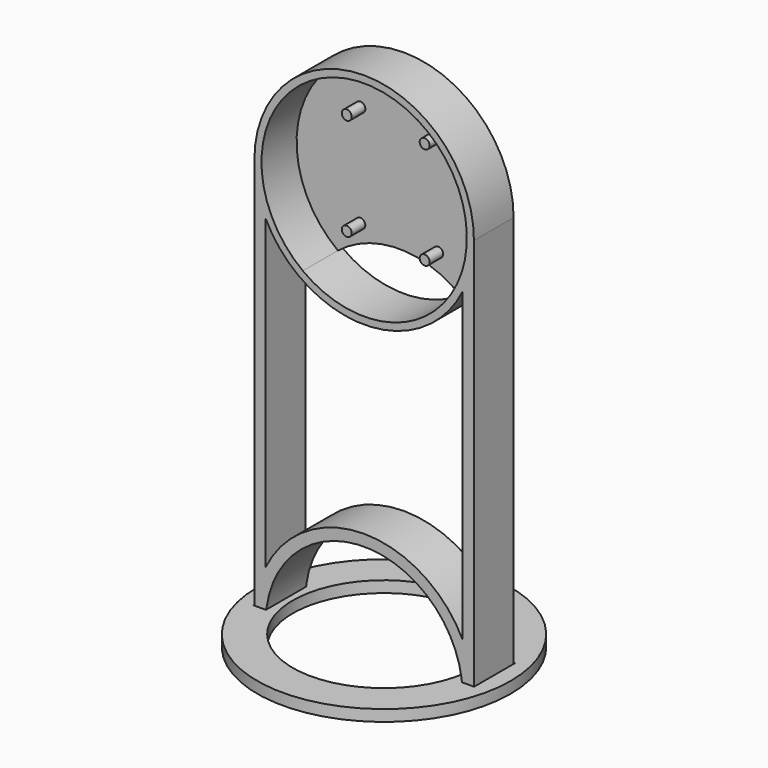
from build123d import *

# Parameters (mm, degrees)
F1_DEPTH    = 14
F0_R        = 1.4
F2_DEPTH    = 1.6
F3_DEPTH    = 6.4
F4_R        = 35.7804971641
F4_W        = 3.6
F4_H        = 14.4
F4_R_2      = 25.7804971641
F5_DEPTH    = 3.2
F8_DEPTH    = 1.6
F9_T1_DEPTH = 3.2
F9_T3_DEPTH = 5.9959172278
F9_T5_DEPTH = 12.5675364253
F10_R       = 0.4


# Not quite as in the source:
# - a fillet or chamfer that OpenCascade refuses, or shapes differently, is made with other operations: its cross-section is extruded or revolved along the edge and cut away or added


with BuildPart() as f1:
    # F0 (on Front) → F1 (new body)
    with BuildSketch(Plane.XZ):
        with BuildLine():
            ThreePointArc((17.3232920146, -23.2573333333), (0, -29), (-17.3232920146, -23.2573333333))
            ThreePointArc((-17.3232920146, -23.2573333333), (-18.1118631329, -23.9097080661), (-18.8758870755, -24.5906666667))
            ThreePointArc((-18.8758870755, -24.5906666667), (0, -31), (18.8758870755, -24.5906666667))
            ThreePointArc((18.8758870755, -24.5906666667), (18.1118631329, -23.9097080661), (17.3232920146, -23.2573333333))
        make_face()
        with BuildLine():
            ThreePointArc((-17.3232920146, -23.2573333333), (-13.0120046799, 25.9169391366), (29, 0))
            ThreePointArc((29, 0), (25.9169391366, -13.0120046799), (17.3232920146, -23.2573333333))
            ThreePointArc((17.3232920146, -23.2573333333), (18.1118631329, -23.9097080661), (18.8758870755, -24.5906666667))
            ThreePointArc((18.8758870755, -24.5906666667), (23.9628460371, -19.6667742602), (27.8, -13.7171425596))
            Line((27.8, -13.7171425596), (27.8, -45))
            Line((27.8, -45), (27.8, -100.2828574404))
            Line((27.8, -100.2828574404), (27.8, -114))
            Line((27.8, -114), (31, -114))
            Line((31, -114), (31, 0))
            ThreePointArc((31, 0), (0, 31), (-31, 0))
            Line((-31, 0), (-31, -114))
            Line((-31, -114), (-27.8, -114))
            Line((-27.8, -114), (-27.8, -100.2828574404))
            Line((-27.8, -100.2828574404), (-27.8, -45))
            Line((-27.8, -45), (-27.8, -13.7171425596))
            ThreePointArc((-27.8, -13.7171425596), (-23.9628460371, -19.6667742602), (-18.8758870755, -24.5906666667))
            ThreePointArc((-18.8758870755, -24.5906666667), (-18.1118631329, -23.9097080661), (-17.3232920146, -23.2573333333))
        make_face()
        with BuildLine():
            ThreePointArc((27.8, -100.2828574404), (0, -83), (-27.8, -100.2828574404))
            Line((-27.8, -100.2828574404), (-27.8, -114))
            ThreePointArc((-27.8, -114), (0, -86.2), (27.8, -114))
            Line((27.8, -114), (27.8, -100.2828574404))
        make_face()
    extrude(amount=F1_DEPTH)

    # F0 (on Front) → F2 (join)
    with BuildSketch(Plane.XZ):
        with BuildLine():
            ThreePointArc((17.3232920146, -23.2573333333), (25.9169391366, -13.0120046799), (29, 0))
            ThreePointArc((29, 0), (-13.0120046799, 25.9169391366), (-17.3232920146, -23.2573333333))
            ThreePointArc((-17.3232920146, -23.2573333333), (0, -17.2), (17.3232920146, -23.2573333333))
        make_face()
        with Locations((-11, -14.45)):
            Circle(F0_R, mode=Mode.SUBTRACT)
        with Locations((-11, 14.45)):
            Circle(F0_R, mode=Mode.SUBTRACT)
        with Locations((11, -14.45)):
            Circle(F0_R, mode=Mode.SUBTRACT)
        with Locations((11, 14.45)):
            Circle(F0_R, mode=Mode.SUBTRACT)
    extrude(amount=F2_DEPTH)

    # F0 (on Front) → F3 (join)
    with BuildSketch(Plane.XZ):
        with Locations((11, -14.45)):
            Circle(F0_R)
        with Locations((-11, -14.45)):
            Circle(F0_R)
        with Locations((-11, 14.45)):
            Circle(F0_R)
        with Locations((11, 14.45)):
            Circle(F0_R)
    extrude(amount=F3_DEPTH)

    # F10
    f10_edges = [f1.edges().sort_by_distance(p)[0] for p in [
        (27.8, -7, -114),
        (31, -7, -114),
        (29.4, -14, -114),
        (29.4, 0, -114),
        (-29.4, 0, -114),
        (-31, -7, -114),
        (-27.8, -7, -114),
        (-29.4, -14, -114),
    ]]
    fillet(f10_edges, radius=F10_R)


with BuildPart() as f5:
    # F4 (on face) → F5 (new body)
    with BuildSketch(Plane(origin=(0, 0, -114), x_dir=(1, 0, 0), z_dir=(0, 0, -1))):
        with Locations((0, 7)):
            Circle(F4_R)
        with Locations((-29.4, 7)):
            Rectangle(F4_W, F4_H, mode=Mode.SUBTRACT)
        with Locations((0, 7)):
            Circle(F4_R_2, mode=Mode.SUBTRACT)
        with Locations((29.4, 7)):
            Rectangle(F4_W, F4_H, mode=Mode.SUBTRACT)
    extrude(amount=-F5_DEPTH)

    # F7 (on offset) → F8 (join, symmetric)
    with BuildSketch(Plane.XZ.offset(-23.2)):
        with BuildLine():
            ThreePointArc((1.5, -107.8606123087), (2.8142494559, -109.076631206), (3.3, -110.8))
            Line((3.3, -110.8), (4.9, -110.8))
            ThreePointArc((4.9, -110.8), (3.9597979746, -107.9138260621), (1.5, -106.1352384841))
            Line((1.5, -106.1352384841), (1.5, -107.8606123087))
        make_face()
        with BuildLine():
            Line((-4.9, -110.8), (-3.3, -110.8))
            ThreePointArc((-3.3, -110.8), (-2.8142494559, -109.076631206), (-1.5, -107.8606123087))
            Line((-1.5, -107.8606123087), (-1.5, -106.1352384841))
            ThreePointArc((-1.5, -106.1352384841), (-3.9597979746, -107.9138260621), (-4.9, -110.8))
        make_face()
    extrude(amount=F8_DEPTH, both=True)

    # F9: fillet of radius 1 on 8 edges, made by hand

    # F9_s2 → F9_t1 (join)
    with BuildSketch(Plane.XZ.offset(-24.8)):
        with BuildLine():
            ThreePointArc((5.814636704, -110.8), (5.1702344715, -110.5646867089), (4.8291050593, -109.9694915254))
            ThreePointArc((4.8291050593, -109.9694915254), (4.8822440942, -110.3832355525), (4.9, -110.8))
            Line((4.9, -110.8), (5.814636704, -110.8))
        make_face()
        with BuildLine():
            ThreePointArc((-5.814636704, -110.8), (-5.1702344715, -110.5646867089), (-4.8291050593, -109.9694915254))
            ThreePointArc((-4.8291050593, -109.9694915254), (-4.8822440942, -110.3832355525), (-4.9, -110.8))
            Line((-4.9, -110.8), (-5.814636704, -110.8))
        make_face()
        with BuildLine():
            ThreePointArc((2.0712315177, -110.8), (2.9182210716, -110.3316095331), (2.9717669602, -109.3652173913))
            ThreePointArc((2.9717669602, -109.3652173913), (3.2168953176, -110.0640757405), (3.3, -110.8))
            Line((3.3, -110.8), (2.0712315177, -110.8))
        make_face()
        with BuildLine():
            ThreePointArc((-2.0712315177, -110.8), (-2.9182210716, -110.3316095331), (-2.9717669602, -109.3652173913))
            ThreePointArc((-2.9717669602, -109.3652173913), (-3.2168953176, -110.0640757405), (-3.3, -110.8))
            Line((-3.3, -110.8), (-2.0712315177, -110.8))
        make_face()
    extrude(amount=F9_T1_DEPTH)

    # F9_s4 → F9_t3 (cut)
    with BuildSketch(Plane.XZ.offset(-26.1979586139)):
        with BuildLine():
            ThreePointArc((1.5, -107.3014288631), (1.6107881724, -107.7589245741), (1.9186046512, -108.1150500577))
            ThreePointArc((1.9186046512, -108.1150500577), (1.7140300704, -107.9800530293), (1.5, -107.8606123087))
            Line((1.5, -107.8606123087), (1.5, -107.3014288631))
        make_face()
        with BuildLine():
            ThreePointArc((-1.5, -107.3014288631), (-1.6107881724, -107.7589245741), (-1.9186046512, -108.1150500577))
            ThreePointArc((-1.9186046512, -108.1150500577), (-1.7140300704, -107.9800530293), (-1.5, -107.8606123087))
            Line((-1.5, -107.8606123087), (-1.5, -107.3014288631))
        make_face()
    extrude(amount=F9_T3_DEPTH, mode=Mode.SUBTRACT)

    # F9_s6 → F9_t5 (cut)
    with BuildSketch(Plane.XZ.offset(-29.4837682127)):
        with BuildLine():
            ThreePointArc((3.141025641, -107.0391546266), (2.0763407271, -106.9008524633), (1.5, -107.8066740906))
            Line((1.5, -107.8066740906), (1.5, -106.1352384841))
            ThreePointArc((1.5, -106.1352384841), (2.3641162933, -106.5080360962), (3.141025641, -107.0391546266))
        make_face()
        with BuildLine():
            ThreePointArc((-3.141025641, -107.0391546266), (-2.0763407271, -106.9008524633), (-1.5, -107.8066740906))
            Line((-1.5, -107.8066740906), (-1.5, -106.1352384841))
            ThreePointArc((-1.5, -106.1352384841), (-2.3641162933, -106.5080360962), (-3.141025641, -107.0391546266))
        make_face()
    extrude(amount=F9_T5_DEPTH, mode=Mode.SUBTRACT)


solid = Compound([f1.part, f5.part])
